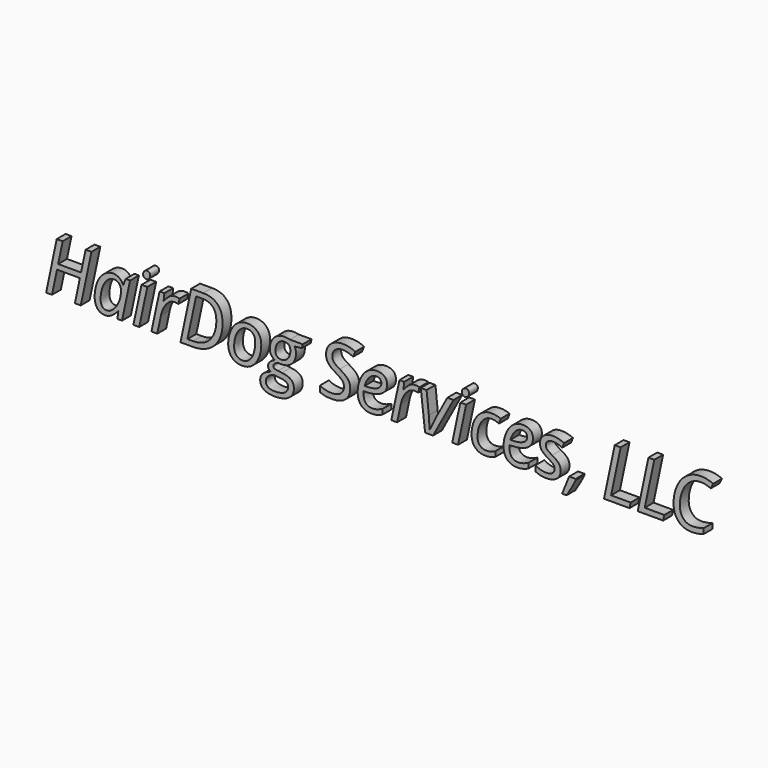
from build123d import *

# Parameters (mm, degrees)
F0_TEXT_SIZE = 40.7578462424
F1_DEPTH     = 6.35


# Not quite as in the source:
# - Text() gives the source's letters only with a copy of the font that has no kerning and outlines rounded to 1/6400 em; it was checked with that copy


with BuildPart() as f1:
    # F0 (on Front) → F1 (new body)
    with BuildSketch(Plane.XZ):
        with Locations((-59.1595806181, 12.4875130132)):
            Text('HairDog Services, LLC', F0_TEXT_SIZE, font='Open Sans', font_style=FontStyle.ITALIC, text_align=(TextAlign.LEFT, TextAlign.BOTTOM))
    extrude(amount=F1_DEPTH)


solid = f1.part
